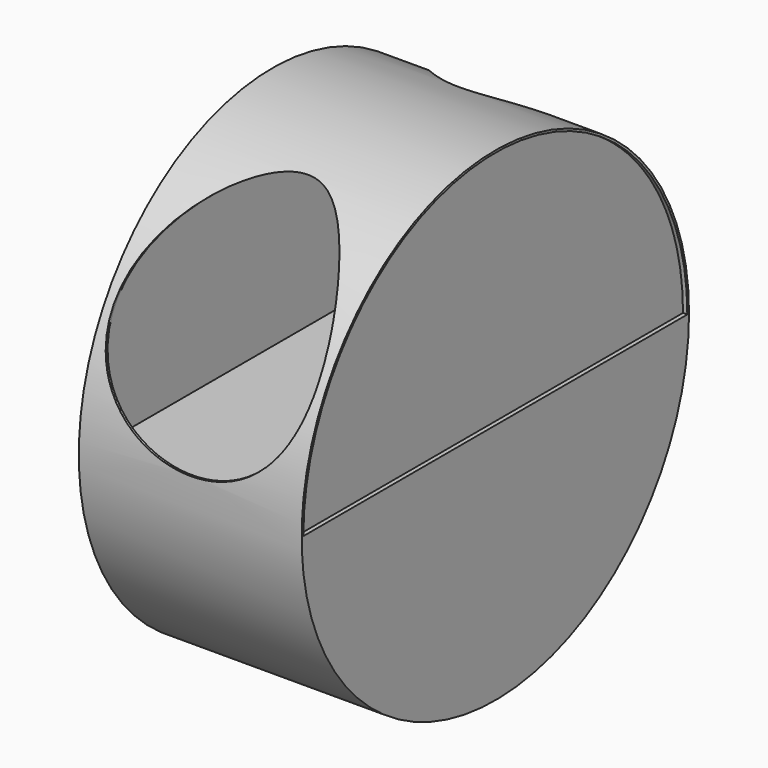
from build123d import *

# Parameters (mm, degrees)
F1_START      = -38.1
F1_DEPTH      = 1.5875
F2_START      = 38.1
F2_DEPTH      = 1.5875
F3_DEPTH      = 38.1
F4_R          = 89.69375
F5_DEPTH      = 39.6875
F5_DEPTH_BACK = 39.6875
F7_DEPTH      = 95.25
F8_START      = 39.6875
F8_DEPTH      = 1.5875
F9_START      = -39.6875
F9_DEPTH      = 1.5875


with BuildPart() as f1:
    # F0 (on Right) → F1 (new body)
    with BuildSketch(Plane.YZ.offset(F1_START)):
        with BuildLine():
            Line((0, 6.35), (88.6729242779, 6.35))
            ThreePointArc((88.6729242779, 6.35), (71.780328059, 52.4480171575), (32.9955678842, 82.55))
            Line((32.9955678842, 82.55), (0, 82.55))
            Line((0, 82.55), (-32.9955678842, 82.55))
            ThreePointArc((-32.9955678842, 82.55), (-71.780328059, 52.4480171575), (-88.6729242779, 6.35))
            Line((-88.6729242779, 6.35), (0, 6.35))
        make_face()
        with BuildLine():
            ThreePointArc((88.8858247627, -1.5875), (88.89645612, -0.793781643), (88.9, 0))
            Line((88.9, 0), (0, 0))
            Line((0, 0), (-88.9, 0))
            ThreePointArc((-88.9, 0), (-88.8963417969, -0.8064831865), (-88.8853674886, -1.6129))
            Line((-88.8853674886, -1.6129), (-3.8579640303, -1.6129))
            Line((-3.8579640303, -1.6129), (-63.9743014562, -61.7292374259))
            ThreePointArc((-63.9743014562, -61.7292374259), (-63.4205753285, -62.2979985634), (-62.8617928475, -62.8617928475))
            ThreePointArc((-62.8617928475, -62.8617928475), (-62.2979985634, -63.4205753285), (-61.7292374259, -63.9743014562))
            Line((-61.7292374259, -63.9743014562), (-1.5875, -3.8325640303))
            Line((-1.5875, -3.8325640303), (-1.5875, -88.8858247627))
            ThreePointArc((-1.5875, -88.8858247627), (-0.793781643, -88.89645612), (0, -88.9))
            ThreePointArc((0, -88.9), (0.793781643, -88.89645612), (1.5875, -88.8858247627))
            Line((1.5875, -88.8858247627), (1.5875, -3.8325640303))
            Line((1.5875, -3.8325640303), (61.7292374259, -63.9743014562))
            ThreePointArc((61.7292374259, -63.9743014562), (62.2979985634, -63.4205753285), (62.8617928475, -62.8617928475))
            ThreePointArc((62.8617928475, -62.8617928475), (63.4205753285, -62.2979985634), (63.9743014562, -61.7292374259))
            Line((63.9743014562, -61.7292374259), (3.8325640303, -1.5875))
            Line((3.8325640303, -1.5875), (88.8858247627, -1.5875))
        make_face()
        Polygon((-1.5875, -1.6129), (-1.6129, -1.6129), (-1.5875, -1.5875), align=None, mode=Mode.SUBTRACT)
        with BuildLine():
            Line((0, 1.5875), (88.8858247627, 1.5875))
            ThreePointArc((88.8858247627, 1.5875), (88.8113038514, 3.9701773533), (88.6729242779, 6.35))
            Line((88.6729242779, 6.35), (0, 6.35))
            Line((0, 6.35), (-88.6729242779, 6.35))
            ThreePointArc((-88.6729242779, 6.35), (-88.8113038514, 3.9701773533), (-88.8858247627, 1.5875))
            Line((-88.8858247627, 1.5875), (0, 1.5875))
        make_face()
        with BuildLine():
            Line((0, 0), (88.9, 0))
            ThreePointArc((88.9, 0), (88.89645612, 0.793781643), (88.8858247627, 1.5875))
            Line((88.8858247627, 1.5875), (0, 1.5875))
            Line((0, 1.5875), (-88.8858247627, 1.5875))
            ThreePointArc((-88.8858247627, 1.5875), (-88.89645612, 0.793781643), (-88.9, 0))
            Line((-88.9, 0), (0, 0))
        make_face()
        with BuildLine():
            Line((0, 82.55), (32.9955678842, 82.55))
            ThreePointArc((32.9955678842, 82.55), (0, 88.9), (-32.9955678842, 82.55))
            Line((-32.9955678842, 82.55), (0, 82.55))
        make_face()
        Polygon((-1.5875, -1.5875), (-1.6129, -1.6129), (-1.5875, -1.6129), align=None)
    extrude(amount=-F1_DEPTH)



with BuildPart() as f2:
    # F0 (on Right) → F2 (new body)
    with BuildSketch(Plane.YZ.offset(F2_START)):
        with BuildLine():
            Line((0, 6.35), (88.6729242779, 6.35))
            ThreePointArc((88.6729242779, 6.35), (71.780328059, 52.4480171575), (32.9955678842, 82.55))
            Line((32.9955678842, 82.55), (0, 82.55))
            Line((0, 82.55), (-32.9955678842, 82.55))
            ThreePointArc((-32.9955678842, 82.55), (-71.780328059, 52.4480171575), (-88.6729242779, 6.35))
            Line((-88.6729242779, 6.35), (0, 6.35))
        make_face()
        with BuildLine():
            ThreePointArc((63.9743014562, -61.7292374259), (82.1328904403, -34.0205571373), (88.8858247627, -1.5875))
            Line((88.8858247627, -1.5875), (3.8325640303, -1.5875))
            Line((3.8325640303, -1.5875), (63.9743014562, -61.7292374259))
        make_face()
        with BuildLine():
            ThreePointArc((88.8858247627, -1.5875), (88.89645612, -0.793781643), (88.9, 0))
            Line((88.9, 0), (0, 0))
            Line((0, 0), (-88.9, 0))
            ThreePointArc((-88.9, 0), (-88.8963417969, -0.8064831865), (-88.8853674886, -1.6129))
            Line((-88.8853674886, -1.6129), (-3.8579640303, -1.6129))
            Line((-3.8579640303, -1.6129), (-63.9743014562, -61.7292374259))
            ThreePointArc((-63.9743014562, -61.7292374259), (-63.4205753285, -62.2979985634), (-62.8617928475, -62.8617928475))
            ThreePointArc((-62.8617928475, -62.8617928475), (-62.2979985634, -63.4205753285), (-61.7292374259, -63.9743014562))
            Line((-61.7292374259, -63.9743014562), (-1.5875, -3.8325640303))
            Line((-1.5875, -3.8325640303), (-1.5875, -88.8858247627))
            ThreePointArc((-1.5875, -88.8858247627), (-0.793781643, -88.89645612), (0, -88.9))
            ThreePointArc((0, -88.9), (0.793781643, -88.89645612), (1.5875, -88.8858247627))
            Line((1.5875, -88.8858247627), (1.5875, -3.8325640303))
            Line((1.5875, -3.8325640303), (61.7292374259, -63.9743014562))
            ThreePointArc((61.7292374259, -63.9743014562), (62.2979985634, -63.4205753285), (62.8617928475, -62.8617928475))
            ThreePointArc((62.8617928475, -62.8617928475), (63.4205753285, -62.2979985634), (63.9743014562, -61.7292374259))
            Line((63.9743014562, -61.7292374259), (3.8325640303, -1.5875))
            Line((3.8325640303, -1.5875), (88.8858247627, -1.5875))
        make_face()
        Polygon((-1.5875, -1.6129), (-1.6129, -1.6129), (-1.5875, -1.5875), align=None, mode=Mode.SUBTRACT)
        with BuildLine():
            Line((0, 1.5875), (88.8858247627, 1.5875))
            ThreePointArc((88.8858247627, 1.5875), (88.8113038514, 3.9701773533), (88.6729242779, 6.35))
            Line((88.6729242779, 6.35), (0, 6.35))
            Line((0, 6.35), (-88.6729242779, 6.35))
            ThreePointArc((-88.6729242779, 6.35), (-88.8113038514, 3.9701773533), (-88.8858247627, 1.5875))
            Line((-88.8858247627, 1.5875), (0, 1.5875))
        make_face()
        with BuildLine():
            Line((0, 0), (88.9, 0))
            ThreePointArc((88.9, 0), (88.89645612, 0.793781643), (88.8858247627, 1.5875))
            Line((88.8858247627, 1.5875), (0, 1.5875))
            Line((0, 1.5875), (-88.8858247627, 1.5875))
            ThreePointArc((-88.8858247627, 1.5875), (-88.89645612, 0.793781643), (-88.9, 0))
            Line((-88.9, 0), (0, 0))
        make_face()
        with BuildLine():
            Line((0, 82.55), (32.9955678842, 82.55))
            ThreePointArc((32.9955678842, 82.55), (0, 88.9), (-32.9955678842, 82.55))
            Line((-32.9955678842, 82.55), (0, 82.55))
        make_face()
        Polygon((-1.5875, -1.5875), (-1.6129, -1.6129), (-1.5875, -1.6129), align=None)
    extrude(amount=F2_DEPTH)


with BuildPart() as f1_1:
    add(f1.part)

    add(f2.part)  # F3 merges F2
    # F0 (on Right) → F3 (join, symmetric)
    with BuildSketch(Plane.YZ):
        with BuildLine():
            ThreePointArc((88.8858247627, -1.5875), (88.89645612, -0.793781643), (88.9, 0))
            Line((88.9, 0), (0, 0))
            Line((0, 0), (-88.9, 0))
            ThreePointArc((-88.9, 0), (-88.8963417969, -0.8064831865), (-88.8853674886, -1.6129))
            Line((-88.8853674886, -1.6129), (-3.8579640303, -1.6129))
            Line((-3.8579640303, -1.6129), (-63.9743014562, -61.7292374259))
            ThreePointArc((-63.9743014562, -61.7292374259), (-63.4205753285, -62.2979985634), (-62.8617928475, -62.8617928475))
            ThreePointArc((-62.8617928475, -62.8617928475), (-62.2979985634, -63.4205753285), (-61.7292374259, -63.9743014562))
            Line((-61.7292374259, -63.9743014562), (-1.5875, -3.8325640303))
            Line((-1.5875, -3.8325640303), (-1.5875, -88.8858247627))
            ThreePointArc((-1.5875, -88.8858247627), (-0.793781643, -88.89645612), (0, -88.9))
            ThreePointArc((0, -88.9), (0.793781643, -88.89645612), (1.5875, -88.8858247627))
            Line((1.5875, -88.8858247627), (1.5875, -3.8325640303))
            Line((1.5875, -3.8325640303), (61.7292374259, -63.9743014562))
            ThreePointArc((61.7292374259, -63.9743014562), (62.2979985634, -63.4205753285), (62.8617928475, -62.8617928475))
            ThreePointArc((62.8617928475, -62.8617928475), (63.4205753285, -62.2979985634), (63.9743014562, -61.7292374259))
            Line((63.9743014562, -61.7292374259), (3.8325640303, -1.5875))
            Line((3.8325640303, -1.5875), (88.8858247627, -1.5875))
        make_face()
        Polygon((-1.5875, -1.6129), (-1.6129, -1.6129), (-1.5875, -1.5875), align=None, mode=Mode.SUBTRACT)
        with BuildLine():
            Line((0, 0), (88.9, 0))
            ThreePointArc((88.9, 0), (88.89645612, 0.793781643), (88.8858247627, 1.5875))
            Line((88.8858247627, 1.5875), (0, 1.5875))
            Line((0, 1.5875), (-88.8858247627, 1.5875))
            ThreePointArc((-88.8858247627, 1.5875), (-88.89645612, 0.793781643), (-88.9, 0))
            Line((-88.9, 0), (0, 0))
        make_face()
        with BuildLine():
            Line((0, 82.55), (32.9955678842, 82.55))
            ThreePointArc((32.9955678842, 82.55), (0, 88.9), (-32.9955678842, 82.55))
            Line((-32.9955678842, 82.55), (0, 82.55))
        make_face()
        Polygon((-1.5875, -1.5875), (-1.6129, -1.6129), (-1.5875, -1.6129), align=None)
    extrude(amount=F3_DEPTH, both=True)


with BuildPart() as f5:
    # F4 (on Right) → F5 (new body, two sides)
    with BuildSketch(Plane.YZ) as f5_sk:
        Circle(F4_R)
        with BuildLine():
            ThreePointArc((-88.9, 0), (0, 88.9), (88.9, 0))
            ThreePointArc((88.9, 0), (0, -88.9), (-88.9, 0))
        make_face(mode=Mode.SUBTRACT)
    extrude(amount=F5_DEPTH)
    extrude(f5_sk.sketch, amount=-F5_DEPTH_BACK)

    # F6 (on Front) → F7 (cut, symmetric)
    with BuildSketch(Plane.XZ):
        with BuildLine():
            ThreePointArc((0, 6.35), (26.9407683632, 17.5092316368), (38.1, 44.45))
            ThreePointArc((38.1, 44.45), (-26.9407683632, 71.3907683632), (0, 6.35))
        make_face()
    extrude(amount=F7_DEPTH, both=True, mode=Mode.SUBTRACT)

    # F4 (on Right) → F8 (join)
    with BuildSketch(Plane.YZ.offset(F8_START)):
        Circle(F4_R)
        with BuildLine():
            ThreePointArc((-88.9, 0), (0, 88.9), (88.9, 0))
            ThreePointArc((88.9, 0), (0, -88.9), (-88.9, 0))
        make_face(mode=Mode.SUBTRACT)
        with BuildLine():
            ThreePointArc((-88.9, 0), (0, -88.9), (88.9, 0))
            Line((88.9, 0), (0, 0))
            Line((0, 0), (-88.9, 0))
        make_face()
    extrude(amount=F8_DEPTH)

    # F4 (on Right) → F9 (join)
    with BuildSketch(Plane.YZ.offset(F9_START)):
        Circle(F4_R)
        with BuildLine():
            ThreePointArc((-88.9, 0), (0, 88.9), (88.9, 0))
            ThreePointArc((88.9, 0), (0, -88.9), (-88.9, 0))
        make_face(mode=Mode.SUBTRACT)
        with BuildLine():
            ThreePointArc((-88.9, 0), (0, -88.9), (88.9, 0))
            Line((88.9, 0), (0, 0))
            Line((0, 0), (-88.9, 0))
        make_face()
    extrude(amount=-F9_DEPTH)


solid = Compound([f1_1.part, f5.part])
